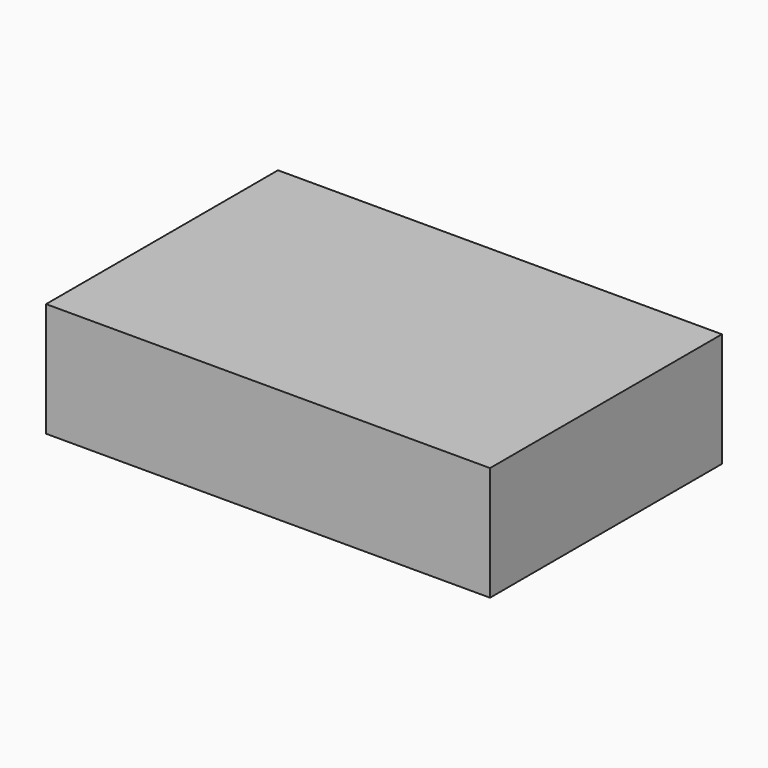
from build123d import *

# Parameters (mm, degrees)
F0_W     = 106.0992144048
F0_H     = 27.2772312164
F1_DEPTH = 69.273641333


# Not quite as in the source:
# - the program builds the solid bodies; features that only make, move or delete a surface that nothing else refers to are left out


with BuildPart() as f1:
    # F0 (on Front) → F1 (new body)
    with BuildSketch(Plane.XZ):
        with Locations((-18.6058748513, 54.5294582844)):
            Rectangle(F0_W, F0_H)
    extrude(amount=F1_DEPTH)


solid = f1.part
